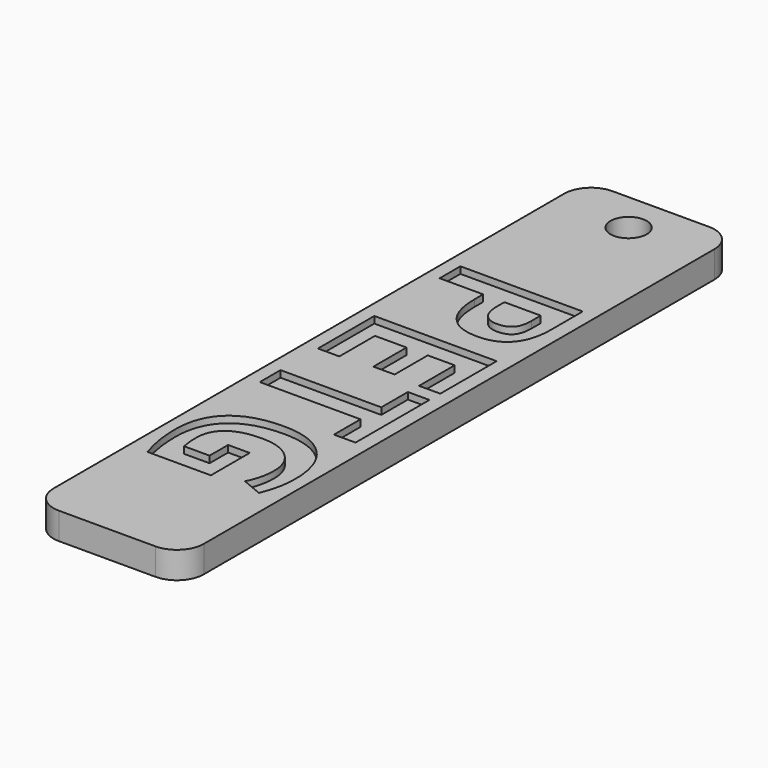
from build123d import *

# Parameters (mm, degrees)
F0_W         = 11.2
F0_H         = 51.6
F0_R         = 1.35
F0_TEXT_SIZE = 12.7777777778
F1_DEPTH     = 2
F2_DEPTH     = 0.5
F3_R         = 2


# Not quite as in the source:
# - Text() gives the source's letters only with a copy of the font that has no kerning and outlines rounded to 1/6400 em; it was checked with that copy


with BuildPart() as f1:
    # F0 (on Top) → F1 (new body)
    with BuildSketch(Plane.XY):
        with Locations((-43.6647401989, 51.1220913022)):
            Rectangle(F0_W, F0_H)
        with BuildLine():
            Line((-44.7528478377, 37.9518656077), (-43.1416499211, 37.9518656077))
            Line((-43.1416499211, 37.9518656077), (-43.1416499211, 34.3321607466))
            Line((-43.1416499211, 34.3321607466), (-47.8714242266, 34.3321607466))
            add(Edge.make_bspline(
                [(-47.8714242266, 34.3321607466), (-48.1589242266, 35.2126294966), (-48.2747228377, 35.9892788022)],
                knots=[0, 0, 0, 1, 1, 1], degree=2))
            add(Edge.make_bspline(
                [(-48.2747228377, 35.9892788022), (-48.3905214489, 36.7659281077), (-48.3905214489, 37.5765183855)],
                knots=[0, 0, 0, 1, 1, 1], degree=2))
            add(Edge.make_bspline(
                [(-48.3905214489, 37.5765183855), (-48.3905214489, 39.6409281077), (-47.17663256, 40.7300340105)],
                knots=[0, 0, 0, 1, 1, 1], degree=2))
            add(Edge.make_bspline(
                [(-47.17663256, 40.7300340105), (-45.9627436711, 41.8191399133), (-43.69069506, 41.8191399133)],
                knots=[0, 0, 0, 1, 1, 1], degree=2))
            add(Edge.make_bspline(
                [(-43.69069506, 41.8191399133), (-41.4825353377, 41.8191399133), (-40.2476829072, 40.55533783)],
                knots=[0, 0, 0, 1, 1, 1], degree=2))
            add(Edge.make_bspline(
                [(-40.2476829072, 40.55533783), (-39.0128304766, 39.2915357466), (-39.0128304766, 37.0534281077)],
                knots=[0, 0, 0, 1, 1, 1], degree=2))
            add(Edge.make_bspline(
                [(-39.0128304766, 37.0534281077), (-39.0128304766, 35.6478725522), (-39.5738547822, 34.3441399133)],
                knots=[0, 0, 0, 1, 1, 1], degree=2))
            Line((-39.5738547822, 34.3441399133), (-41.12116381, 34.9870218577))
            add(Edge.make_bspline(
                [(-41.12116381, 34.9870218577), (-40.6220318655, 35.9852857466), (-40.6220318655, 37.0654072744)],
                knots=[0, 0, 0, 1, 1, 1], degree=2))
            add(Edge.make_bspline(
                [(-40.6220318655, 37.0654072744), (-40.6220318655, 38.3192267188), (-41.4645665877, 39.0739142188)],
                knots=[0, 0, 0, 1, 1, 1], degree=2))
            add(Edge.make_bspline(
                [(-41.4645665877, 39.0739142188), (-42.30710131, 39.8286017188), (-43.7286290877, 39.8286017188)],
                knots=[0, 0, 0, 1, 1, 1], degree=2))
            add(Edge.make_bspline(
                [(-43.7286290877, 39.8286017188), (-45.2140457544, 39.8286017188), (-45.9966846433, 39.2206590105)],
                knots=[0, 0, 0, 1, 1, 1], degree=2))
            add(Edge.make_bspline(
                [(-45.9966846433, 39.2206590105), (-46.7793235322, 38.6127163022), (-46.7793235322, 37.4527336633)],
                knots=[0, 0, 0, 1, 1, 1], degree=2))
            add(Edge.make_bspline(
                [(-46.7793235322, 37.4527336633), (-46.7793235322, 36.8457892188), (-46.65553881, 36.2228725522)],
                knots=[0, 0, 0, 1, 1, 1], degree=2))
            Line((-46.65553881, 36.2228725522), (-44.7528478377, 36.2228725522))
            Line((-44.7528478377, 36.2228725522), (-44.7528478377, 37.9518656077))
        make_face(mode=Mode.SUBTRACT)
        Polygon((-40.7518061711, 45.2930982466), (-48.2647401989, 45.2930982466), (-48.2647401989, 47.2277336633), (-40.7518061711, 47.2277336633), (-40.7518061711, 49.7054246355), (-39.1426047822, 49.7054246355), (-39.1426047822, 42.8174038022), (-40.7518061711, 42.8174038022), align=None, mode=Mode.SUBTRACT)
        Polygon((-46.6675179766, 50.7156676911), (-48.2647401989, 50.7156676911), (-48.2647401989, 55.9685322744), (-39.1426047822, 55.9685322744), (-39.1426047822, 50.7156676911), (-40.7278478377, 50.7156676911), (-40.7278478377, 54.0338968577), (-42.7303651989, 54.0338968577), (-42.7303651989, 50.9452683855), (-44.3156082544, 50.9452683855), (-44.3156082544, 54.0338968577), (-46.6675179766, 54.0338968577), align=None, mode=Mode.SUBTRACT)
        with BuildLine():
            add(Edge.make_bspline(
                [(-39.8573617266, 58.5550340105), (-40.5721186711, 57.6915357466), (-41.9876568655, 57.6915357466)],
                knots=[0, 0, 0, 1, 1, 1], degree=2))
            add(Edge.make_bspline(
                [(-41.9876568655, 57.6915357466), (-43.4610943655, 57.6915357466), (-44.2407384627, 58.6119350522)],
                knots=[0, 0, 0, 1, 1, 1], degree=2))
            add(Edge.make_bspline(
                [(-44.2407384627, 58.6119350522), (-45.02038256, 59.5323343577), (-45.02038256, 61.2293829688)],
                knots=[0, 0, 0, 1, 1, 1], degree=2))
            Line((-45.02038256, 61.2293829688), (-45.02038256, 62.0579419966))
            Line((-45.02038256, 62.0579419966), (-48.2647401989, 62.0579419966))
            Line((-48.2647401989, 62.0579419966), (-48.2647401989, 63.9925774133))
            Line((-48.2647401989, 63.9925774133), (-39.1426047822, 63.9925774133))
            Line((-39.1426047822, 63.9925774133), (-39.1426047822, 61.0796433855))
            add(Edge.make_bspline(
                [(-39.1426047822, 61.0796433855), (-39.1426047822, 59.4185322744), (-39.8573617266, 58.5550340105)],
                knots=[0, 0, 0, 1, 1, 1], degree=2))
        make_face(mode=Mode.SUBTRACT)
        with Locations((-43.6647401989, 73.9220913022)):
            Circle(F0_R, mode=Mode.SUBTRACT)
        with BuildLine():
            Line((-40.7278478377, 62.0579419966), (-43.4351395044, 62.0579419966))
            Line((-43.4351395044, 62.0579419966), (-43.4351395044, 61.4210496355))
            add(Edge.make_bspline(
                [(-43.4351395044, 61.4210496355), (-43.4351395044, 60.5305982466), (-43.0827523516, 60.08736908)],
                knots=[0, 0, 0, 1, 1, 1], degree=2))
            add(Edge.make_bspline(
                [(-43.0827523516, 60.08736908), (-42.7303651989, 59.6441399133), (-42.0575353377, 59.6441399133)],
                knots=[0, 0, 0, 1, 1, 1], degree=2))
            add(Edge.make_bspline(
                [(-42.0575353377, 59.6441399133), (-41.3767193655, 59.6441399133), (-41.0522836016, 60.01549408)],
                knots=[0, 0, 0, 1, 1, 1], degree=2))
            add(Edge.make_bspline(
                [(-41.0522836016, 60.01549408), (-40.7278478377, 60.3868482466), (-40.7278478377, 61.1794697744)],
                knots=[0, 0, 0, 1, 1, 1], degree=2))
            Line((-40.7278478377, 61.1794697744), (-40.7278478377, 62.0579419966))
        make_face()
        with Locations(Location((-48.2647401989, 65.1405808855), (0, 0, -90))):
            Text('PETG', F0_TEXT_SIZE, font='Open Sans', font_style=FontStyle.BOLD, text_align=(TextAlign.LEFT, TextAlign.BOTTOM))
    extrude(amount=-F1_DEPTH)

    # F0 (on Top) → F2 (cut)
    with BuildSketch(Plane.XY):
        with Locations(Location((-48.2647401989, 65.1405808855), (0, 0, -90))):
            Text('PETG', F0_TEXT_SIZE, font='Open Sans', font_style=FontStyle.BOLD, text_align=(TextAlign.LEFT, TextAlign.BOTTOM))
    extrude(amount=-F2_DEPTH, mode=Mode.SUBTRACT)

    # F3
    f3_edges = [f1.edges().sort_by_distance(p)[0] for p in [
        (-49.26474, 76.922091, -1),
        (-38.06474, 76.922091, -1),
        (-38.06474, 25.322091, -1),
        (-49.26474, 25.322091, -1),
    ]]
    fillet(f3_edges, radius=F3_R)


solid = f1.part
